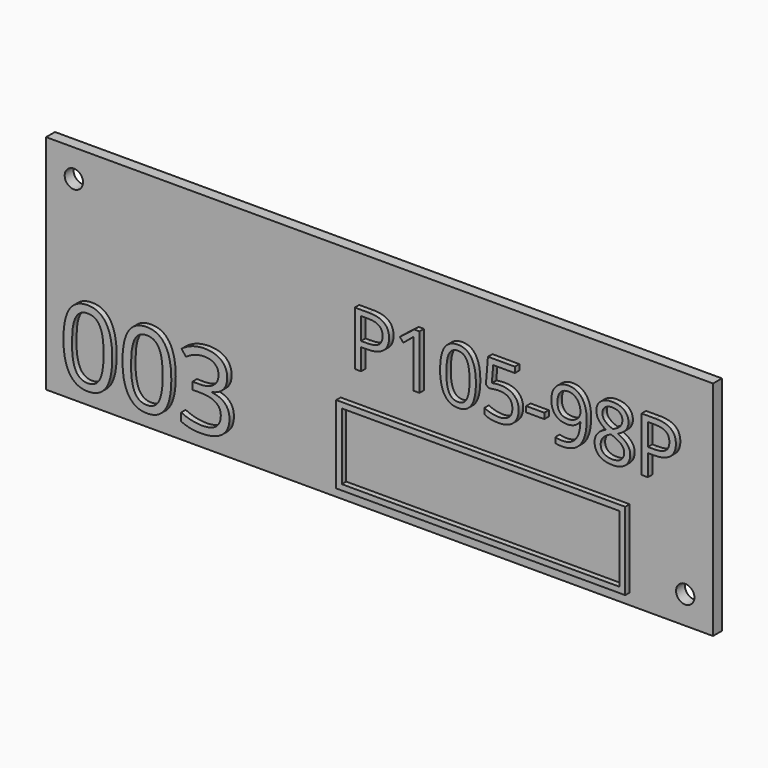
from build123d import *

# Parameters (mm, degrees)
F0_W         = 120
F0_H         = 40
F1_DEPTH     = 2
F3_D         = 3.3
F4_TEXT_SIZE = 13.6426617401
F5_DEPTH     = 1
F6_TEXT_SIZE = 18.5894526641
F7_DEPTH     = 1
F8_W         = 52
F8_H         = 14
F8_W_2       = 49.99999962
F8_H_2       = 11.99999962
F9_DEPTH     = 1


# Not quite as in the source:
# - Text() gives the source's letters only with a copy of the font that has no kerning and outlines rounded to 1/6400 em; it was checked with that copy


with BuildPart() as f1:
    # F0 (on Front) → F1 (new body)
    with BuildSketch(Plane.XZ):
        Rectangle(F0_W, F0_H)
    extrude(amount=F1_DEPTH)

    # F3 (through all)
    with Locations(Plane.XZ.offset(2)):
        with Locations((-55, 15), (55, -15)):
            Hole(F3_D / 2)

    # F4 (on face) → F5 (join)
    with BuildSketch(Plane.XZ.offset(2)):
        with Locations((-5, 2)):
            Text('P105-98P', F4_TEXT_SIZE, font='Open Sans', text_align=(TextAlign.LEFT, TextAlign.BOTTOM))
    extrude(amount=F5_DEPTH)

    # F6 (on face) → F7 (join)
    with BuildSketch(Plane.XZ.offset(2)):
        with Locations((-57, -17)):
            Text('003', F6_TEXT_SIZE, font='Open Sans', text_align=(TextAlign.LEFT, TextAlign.BOTTOM))
    extrude(amount=F7_DEPTH)

    # F8 (on face) → F9 (join)
    with BuildSketch(Plane.XZ.offset(2)):
        with Locations((19, -11)):
            Rectangle(F8_W, F8_H)
        with Locations((19, -11)):
            Rectangle(F8_W_2, F8_H_2, mode=Mode.SUBTRACT)
    extrude(amount=F9_DEPTH)


solid = f1.part
